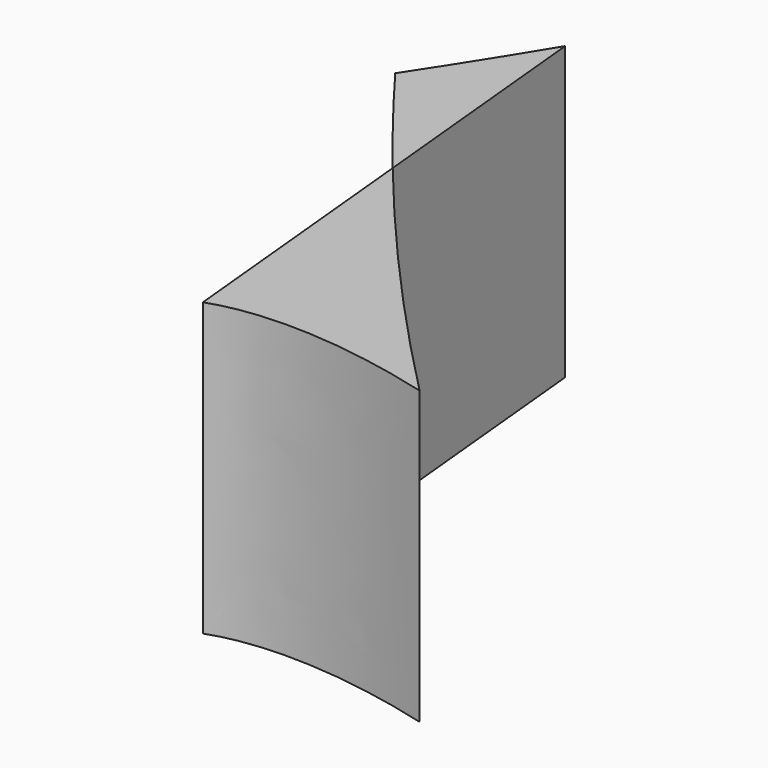
from build123d import *

# Parameters (mm, degrees)
F1_DEPTH = 6.35
F2_DEPTH = 6.35


with BuildPart() as f1:
    # F0 (on Top) → F1 (new body)
    with BuildSketch(Plane.XY):
        with BuildLine():
            ThreePointArc((78.4370391826, -86.7501992629), (75.624927239, -83.7578477701), (72.9588367307, -80.6346919236))
            Line((72.9588367307, -80.6346919236), (73.526725173, -86.5121111274))
            add(Edge.make_bspline(
                [(78.4370391826, -86.7501992629), (76.8349189463, -86.3184887646), (74.8358563915, -86.03503847), (73.526725173, -86.5121111274)],
                knots=[0.7001399432, 0.7001399432, 0.7001399432, 0.7001399432, 0.7108428606, 0.7108428606, 0.7108428606, 0.7108428606], degree=3))
        make_face()
    extrude(amount=F1_DEPTH)


with BuildPart() as f2:
    # F0 (on Top) → F2 (new body)
    with BuildSketch(Plane.XY):
        with BuildLine():
            Line((72.9588367307, -80.6346919236), (72.4430223898, -75.2962189308))
            ThreePointArc((72.4430223898, -75.2962189308), (71.6393776624, -76.5966527102), (70.8115200426, -77.8818081965))
            ThreePointArc((70.8115200426, -77.8818081965), (71.8712093435, -79.2691462556), (72.9588367307, -80.6346919236))
        make_face()
    extrude(amount=F2_DEPTH)


solid = Compound([f1.part, f2.part])
